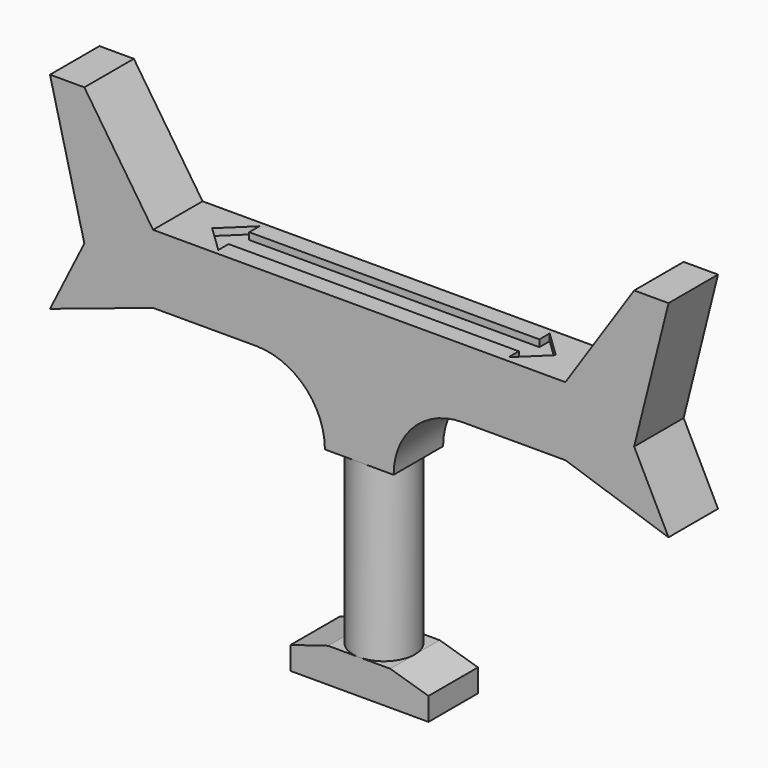
from build123d import *

# Parameters (mm, degrees)
F1_DEPTH  = 9
F2_W      = 42.22
F2_H      = 1.875
F3_DEPTH  = 1
F4_W      = 10
F4_H      = 9
F5_DEPTH  = 10
F6_R      = 9.99999
F7_R      = 4.5
F8_DEPTH  = 25
F10_DEPTH = 5
F12_DEPTH = 25


# Not quite as in the source:
# - a fillet or chamfer is up to 0.001 mm smaller than in the source, because OpenCascade refuses the exact size


with BuildPart() as f1:
    # F0 (on Front) → F1 (new body)
    with BuildSketch(Plane.XZ):
        Polygon((30, 3.7309644414), (0, 3.7309644414), (-30, 3.7309644414), (-40, 18.7309644414), (-45, 18.7309644414), (-40, -1.2690355586), (-45, -11.2690355586), (-30, -6.2690355586), (0, -6.2690355586), (30, -6.2690355586), (45, -11.2690355586), (40, -1.2690355586), (45, 18.7309644414), (40, 18.7309644414), align=None)
    extrude(amount=F1_DEPTH)

    # F2 (on face) → F3 (cut)
    with BuildSketch(Plane.XY.offset(3.7309644414)):
        Polygon((21.11, -8.25), (25, -4.5), (21.11, -4.5), (21.11, -6.375), align=None)
        Polygon((21.11, -4.5), (25, -4.5), (21.11, -0.75), (21.11, -2.625), align=None)
        with Locations((0, -5.4375)):
            Rectangle(F2_W, F2_H)
        with Locations((0, -3.5625)):
            Rectangle(F2_W, F2_H)
        Polygon((-21.11, -6.375), (-21.11, -4.5), (-25, -4.5), (-21.11, -8.25), align=None)
        Polygon((-25, -4.5), (-21.11, -4.5), (-21.11, -2.625), (-21.11, -0.75), align=None)
    extrude(amount=-F3_DEPTH, mode=Mode.SUBTRACT)

    # F4 (on face) → F5 (join)
    with BuildSketch(Plane(origin=(0, 0, -6.2690355586), x_dir=(1, 0, 0), z_dir=(0, 0, -1))):
        with Locations((0, 4.5)):
            Rectangle(F4_W, F4_H)
    extrude(amount=F5_DEPTH)

    # F6 (radius 10 in the source; OpenCascade refuses exactly that, so slightly less here)
    f6_edges = [f1.edges().sort_by_distance(p)[0] for p in [
        (5, -4.5, -6.269036),
        (-5, -4.5, -6.269036),
    ]]
    fillet(f6_edges, radius=F6_R)

    # F7 (on face) → F8 (join)
    with BuildSketch(Plane(origin=(0, 0, -16.2690355586), x_dir=(1, 0, 0), z_dir=(0, 0, -1))):
        with Locations((0, 4.5)):
            Circle(F7_R)
    extrude(amount=F8_DEPTH)

    # F9 (on face) → F10 (join)
    with BuildSketch(Plane(origin=(0, 0, -41.2690355586), x_dir=(1, 0, 0), z_dir=(0, 0, -1))):
        Polygon((-10, 0), (0, 0), (10.0785335526, 0), (10.0785335526, 9), (0, 9), (-10, 9), align=None)
    extrude(amount=F10_DEPTH)

    # F11 (on face) → F12 (cut)
    with BuildSketch(Plane.XZ.offset(9)):
        Polygon((-10, -41.2690355586), (-10, -42.9390355586), (-4.5407158323, -41.2690355586), align=None)
        Polygon((10.0785335526, -41.2690355586), (4.5102024451, -41.2690355586), (10.0785335526, -42.9390355586), align=None)
    extrude(amount=-F12_DEPTH, mode=Mode.SUBTRACT)


solid = f1.part
